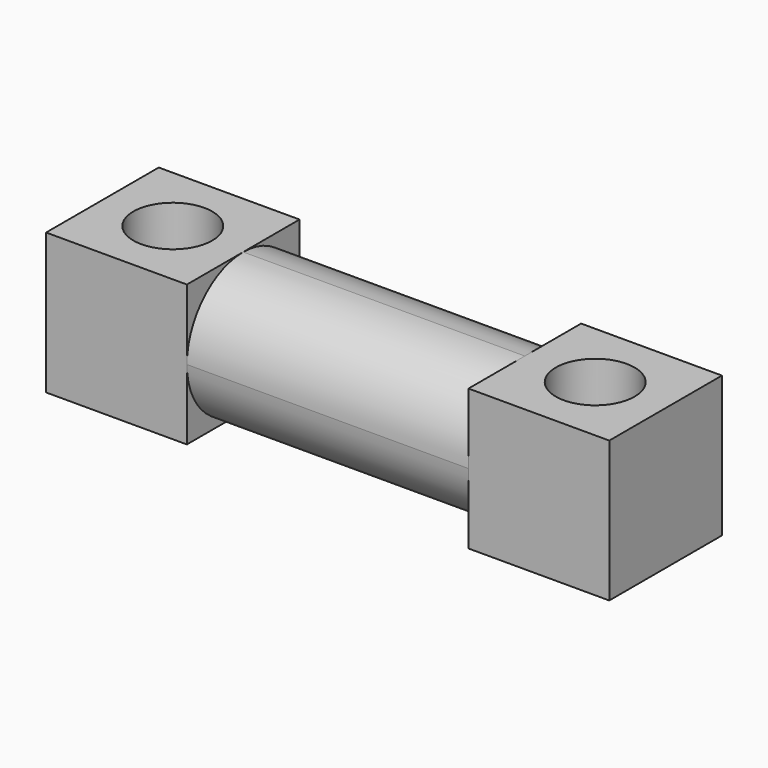
from build123d import *

# Parameters (mm, degrees)
F0_W     = 25.4
F0_H     = 25.4
F0_R     = 7.112
F1_DEPTH = 25.4
F3_DEPTH = 76.2
F4_R     = 7.112
F4_W     = 50.8
F4_H     = 25.4
F5_DEPTH = 25.401
F6_DEPTH = 50.8
F7_R     = 7.112
F8_DEPTH = 148


# Not quite as in the source:
# - an extrude ends at something that could not be found from the text; its depth is read off the source's solid


with BuildPart() as f1:
    # F0 (on Top) → F1 (new body)
    with BuildSketch(Plane.XY):
        Rectangle(F0_W, F0_H)
        Circle(F0_R, mode=Mode.SUBTRACT)
    extrude(amount=F1_DEPTH)

    # F2 (on face) → F3 (join)
    with BuildSketch(Plane(origin=(-12.7, 0, 0), x_dir=(0, -1, 0), z_dir=(-1, 0, 0))):
        with BuildLine():
            ThreePointArc((-12.7, 12.7), (-8.9802561211, 21.6802561211), (0, 25.4))
            Line((0, 25.4), (-12.7, 25.4))
            Line((-12.7, 25.4), (-12.7, 12.7))
        make_face()
        with BuildLine():
            ThreePointArc((0, 25.4), (8.9802561211, 21.6802561211), (12.7, 12.7))
            Line((12.7, 12.7), (12.7, 25.4))
            Line((12.7, 25.4), (0, 25.4))
        make_face()
        with BuildLine():
            Line((12.7, 0), (12.7, 12.7))
            ThreePointArc((12.7, 12.7), (8.9802561211, 3.7197438789), (0, 0))
            Line((0, 0), (12.7, 0))
        make_face()
        with BuildLine():
            Line((-12.7, 0), (0, 0))
            ThreePointArc((0, 0), (-8.9802561211, 3.7197438789), (-12.7, 12.7))
            Line((-12.7, 12.7), (-12.7, 0))
        make_face()
        with BuildLine():
            ThreePointArc((0, 0), (8.9802561211, 3.7197438789), (12.7, 12.7))
            ThreePointArc((12.7, 12.7), (8.9802561211, 21.6802561211), (0, 25.4))
            ThreePointArc((0, 25.4), (-8.9802561211, 21.6802561211), (-12.7, 12.7))
            ThreePointArc((-12.7, 12.7), (-8.9802561211, 3.7197438789), (0, 0))
        make_face()
    extrude(amount=F3_DEPTH)

    # F4 (on face) → F5 (cut, through all)
    with BuildSketch(Plane.XY.offset(25.4)):
        with Locations((-76.2, 0)):
            Circle(F4_R)
        with Locations((-38.1, 0)):
            Rectangle(F4_W, F4_H)
    extrude(amount=-F5_DEPTH, mode=Mode.SUBTRACT)

    # F2 (on face) → F6 (join, through all)
    with BuildSketch(Plane(origin=(-12.7, 0, 0), x_dir=(0, -1, 0), z_dir=(-1, 0, 0))):
        with BuildLine():
            ThreePointArc((0, 0), (8.9802561211, 3.7197438789), (12.7, 12.7))
            ThreePointArc((12.7, 12.7), (8.9802561211, 21.6802561211), (0, 25.4))
            ThreePointArc((0, 25.4), (-8.9802561211, 21.6802561211), (-12.7, 12.7))
            ThreePointArc((-12.7, 12.7), (-8.9802561211, 3.7197438789), (0, 0))
        make_face()
    extrude(amount=F6_DEPTH)

    # F7 (on face) → F8 (cut, through all)
    with BuildSketch(Plane(origin=(0, 0, 0), x_dir=(1, 0, 0), z_dir=(0, 0, -1))):
        Polygon((-63.5, 0), (-63.5, 12.7), (-88.9, 12.7), (-88.9, -12.7), (-63.5, -12.7), align=None)
        with Locations((-76.2, 0)):
            Circle(F7_R, mode=Mode.SUBTRACT)
    extrude(amount=F8_DEPTH, mode=Mode.SUBTRACT)


solid = f1.part
